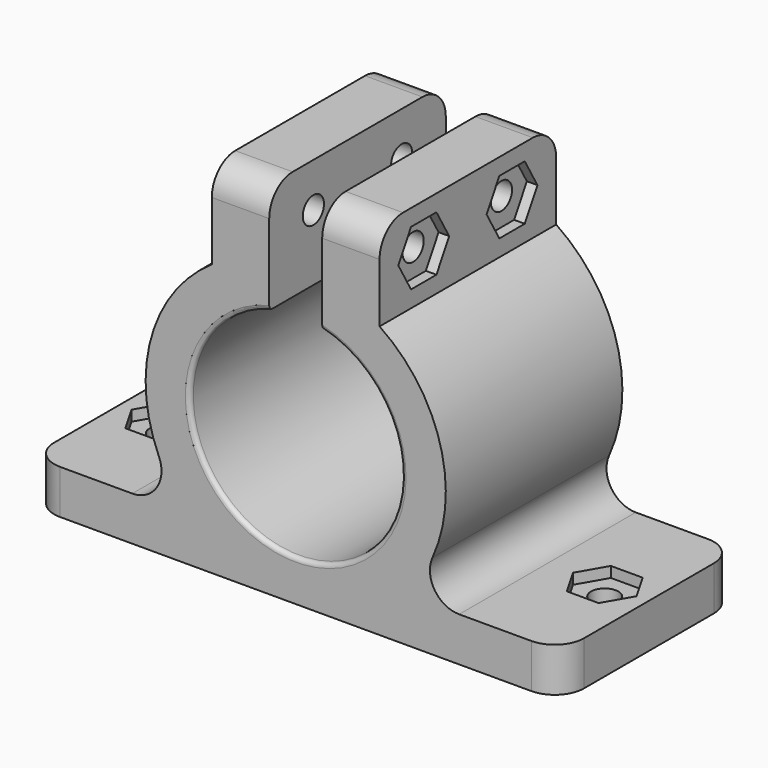
from build123d import *

# Parameters (mm, degrees)
F1_DEPTH  = 25
F2_R      = 1.55
F3_DEPTH  = 25
F4_R      = 1.5
F5_DEPTH  = 25
F6_R      = 3.3134143982
F9_DEPTH  = 1.2
F8_R      = 1.5
F10_DEPTH = 1.2
F12_DEPTH = 1.2
F13_R     = 0.5


# Not quite as in the source:
# - ends of sketch curves that miss each other by under 0.0002 mm in the source are joined


with BuildPart() as f1:
    # F0 (on Front) → F1 (new body)
    with BuildSketch(Plane.XZ):
        with BuildLine():
            Line((-30, -27.2712218283), (30, -27.271222222))
            Line((30, -27.271222222), (30, -22.271222222))
            Line((30, -22.271222222), (12.3570600307, -22.2712218283))
            ThreePointArc((12.3570600307, -22.2712218283), (16.8965495982, -8.7237267257), (9.5007861894, 3.5010134632))
            Line((9.5007861894, 3.5010134632), (9.5007861894, 13.5010134632))
            Line((9.5007861894, 13.5010134632), (3, 13.5010134632))
            Line((3, 13.5010134632), (3, 6.1368714524))
            Line((3, 6.1368714524), (3, 4.8868714524))
            Line((3, 4.8868714524), (3, 1.0226200218))
            ThreePointArc((3, 1.0226200218), (0, -22.5963300169), (-3, 1.0226200218))
            Line((-3, 1.0226200218), (-3, 4.8868714524))
            Line((-3, 4.8868714524), (-3, 13.5010134632))
            Line((-3, 13.5010134632), (-9.5007861894, 13.5010134632))
            Line((-9.5007861894, 13.5010134632), (-9.5007861894, 3.5010134632))
            ThreePointArc((-9.5007861894, 3.5010134632), (-16.8965495982, -8.7237267257), (-12.3570600307, -22.2712218283))
            Line((-12.3570600307, -22.2712218283), (-30, -22.2712218283))
            Line((-30, -22.2712218283), (-30, -27.2712218283))
        make_face()
    extrude(amount=F1_DEPTH)

    # F2 (on face) → F3 (cut)
    with BuildSketch(Plane.XY.offset(-22.2712218283)):
        with Locations((-25, -12.5)):
            Circle(F2_R)
        with Locations((25, -12.5)):
            Circle(F2_R)
    extrude(amount=-F3_DEPTH, mode=Mode.SUBTRACT)

    # F4 (on face) → F5 (cut)
    with BuildSketch(Plane.YZ.offset(9.5007861894)):
        with Locations((-18.75, 8.5010134632)):
            Circle(F4_R)
        with Locations((-6.25, 8.5010134632)):
            Circle(F4_R)
    extrude(amount=-F5_DEPTH, mode=Mode.SUBTRACT)

    # F6
    f6_edges = [f1.edges().sort_by_distance(p)[0] for p in [
        (-6.250393, -25, 13.501013),
        (6.250393, -25, 13.501013),
        (-6.250393, 0, 13.501013),
        (6.250393, 0, 13.501013),
        (30, -25, -24.771222),
        (30, 0, -24.771222),
        (-30, 0, -24.771222),
        (-30, -25, -24.771222),
        (12.35706, -12.5, -22.271222),
        (-12.35706, -12.5, -22.271222),
    ]]
    fillet(f6_edges, radius=F6_R)

    # F7 (on face) → F9 (cut)
    with BuildSketch(Plane.YZ.offset(9.5007861894)):
        Polygon((-20.55, 5.3833220096), (-16.95, 5.3833220096), (-15.15, 8.5010134632), (-16.95, 11.6187049168), (-20.55, 11.6187049168), (-22.35, 8.5010134632), align=None)
        Polygon((-4.45, 11.6187049168), (-8.05, 11.6187049168), (-9.85, 8.5010134632), (-8.05, 5.3833220096), (-4.45, 5.3833220096), (-2.65, 8.5010134632), align=None)
    extrude(amount=-F9_DEPTH, mode=Mode.SUBTRACT)

    # F8 (on face) → F10 (cut)
    with BuildSketch(Plane(origin=(-9.5007861894, 0, 0), x_dir=(0, -1, 0), z_dir=(-1, 0, 0))):
        Polygon((4.45, 5.3833220096), (8.05, 5.3833220096), (9.85, 8.5010134632), (8.05, 11.6187049168), (4.45, 11.6187049168), (2.65, 8.5010134632), align=None)
        with Locations((6.25, 8.5010134632)):
            Circle(F8_R, mode=Mode.SUBTRACT)
        Polygon((20.55, 11.6187049168), (16.95, 11.6187049168), (15.15, 8.5010134632), (16.95, 5.3833220096), (20.55, 5.3833220096), (22.35, 8.5010134632), align=None)
        with Locations((18.75, 8.5010134632)):
            Circle(F8_R, mode=Mode.SUBTRACT)
    extrude(amount=-F10_DEPTH, mode=Mode.SUBTRACT)

    # F11 (on face) → F12 (cut)
    with BuildSketch(Plane.XY.offset(-22.2712218283)):
        Polygon((26.8, -9.3823085464), (23.2, -9.3823085464), (21.4, -12.5), (23.2, -15.6176914536), (26.8, -15.6176914536), (28.6, -12.5), align=None)
        Polygon((-23.2, -15.6176914536), (-21.4, -12.5), (-23.2, -9.3823085464), (-26.8, -9.3823085464), (-28.6, -12.5), (-26.8, -15.6176914536), align=None)
    extrude(amount=-F12_DEPTH, mode=Mode.SUBTRACT)

    # F13
    f13_edges = [f1.edges().sort_by_distance(p)[0] for p in [
        (0, 0, -22.59633),
        (0, -25, -22.59633),
    ]]
    fillet(f13_edges, radius=F13_R)


solid = f1.part
